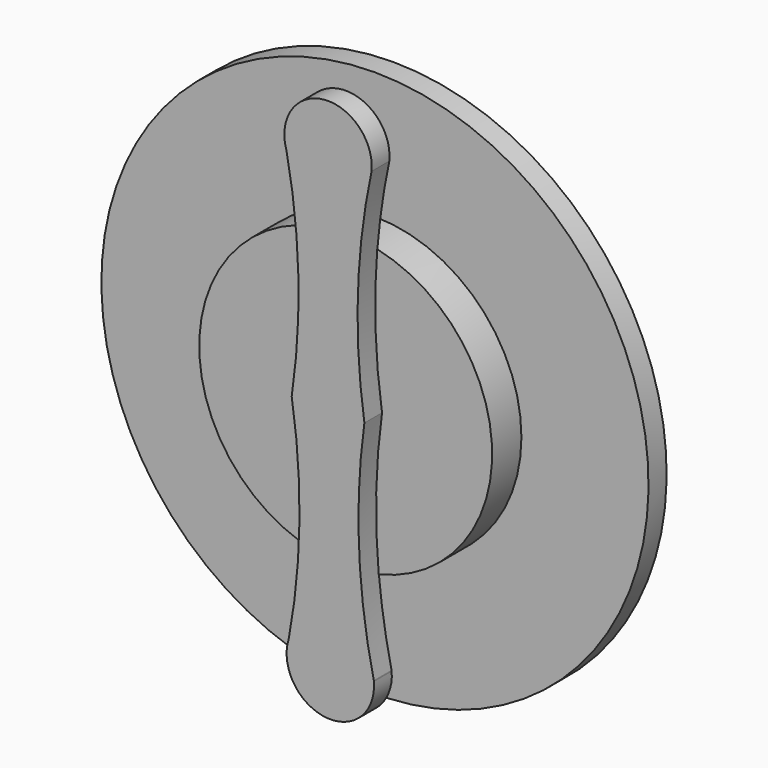
from build123d import *
from build123d import SkipClean  # not in build123d's __all__

# Parameters (mm, degrees)
F3_DEPTH = 25
F4_DEPTH = 9.7316764295
F5_R     = 2.7549652458
F6_DEPTH = 8.4777977318


with BuildPart() as f1:
    # F0 (on Right) → F1 (revolve)
    with BuildSketch(Plane.YZ):
        Polygon((0, 6.1400169507), (0, 8.2560488954), (0, 19.687499851), (-8.4777977318, 19.687499851), (-8.4777977318, 14.3298944458), (-25.8282721043, 14.3298944458), (-25.8282721043, 100.0597700477), (-35.5599485338, 100.0597700477), (-35.5599485338, 6.1400169507), align=None)
    revolve(axis=Axis((0, -24.406015873, 0), (0, -1, 0)))

    # F2 (on face) → F3 (cut)
    with BuildSketch(Plane.XZ.offset(35.5599485338)):
        with BuildLine():
            ThreePointArc((100.0597700477, 0), (77.1925232945, 63.6653118222), (19.0427553675, 98.2310085971))
            ThreePointArc((19.0427553675, 98.2310085971), (13.0501122552, 49.3824410014), (15.9002061052, 0.2502591582))
            ThreePointArc((15.9002061052, 0.2502591582), (13.5409533991, -48.9079370484), (20.0211640805, -97.6942178777))
            ThreePointArc((20.0211640805, -97.6942178777), (20.0382067589, -97.8618404932), (20.0537724887, -98.0296067062))
            ThreePointArc((20.0537724887, -98.0296067062), (77.5194602851, -63.2668227359), (100.0597700477, 0))
        make_face()
        with BuildLine():
            ThreePointArc((-18.1994950958, 94.1649181676), (-18.6134156028, 96.1995622705), (-19.0427553675, 98.2310085971))
            ThreePointArc((-19.0427553675, 98.2310085971), (-18.7317798871, 96.1750148827), (-18.1994950958, 94.1649181676))
        make_face()
        with BuildLine():
            ThreePointArc((-18.1994950958, 94.1649181676), (-18.7317798871, 96.1750148827), (-19.0427553675, 98.2310085971))
            ThreePointArc((-19.0427553675, 98.2310085971), (-100.058591646, -0.4856128205), (-18.0883946868, -98.4112166353))
            ThreePointArc((-18.0883946868, -98.4112166353), (-18.0761635611, -98.2428461722), (-18.0624471565, -98.0745901959))
            ThreePointArc((-18.0624471565, -98.0745901959), (-17.7720210603, -96.0155932105), (-17.2598383027, -94.0002806477))
            ThreePointArc((-17.2598383027, -94.0002806477), (-12.518858774, -47.0123005144), (-15.9239394561, 0.0913361759))
            ThreePointArc((-15.9239394561, 0.0913361759), (-12.9894678609, 47.2266312356), (-18.1994950958, 94.1649181676))
        make_face()
    extrude(amount=-F3_DEPTH, mode=Mode.SUBTRACT)

    # F2 (on face) → F4 (join, through all)
    with BuildSketch(Plane.XZ.offset(35.5599485338)):
        with BuildLine():
            ThreePointArc((15.9002061052, 0.2502591582), (13.0501122552, 49.3824410014), (19.0427553675, 98.2310085971))
            ThreePointArc((19.0427553675, 98.2310085971), (0, 119.1901359728), (-19.0427553675, 98.2310085971))
            ThreePointArc((-19.0427553675, 98.2310085971), (-18.6134156028, 96.1995622705), (-18.1994950958, 94.1649181676))
            ThreePointArc((-18.1994950958, 94.1649181676), (-12.9894678609, 47.2266312356), (-15.9239394561, 0.0913361759))
            ThreePointArc((-15.9239394561, 0.0913361759), (-12.518858774, -47.0123005144), (-17.2598383027, -94.0002806477))
            ThreePointArc((-17.2598383027, -94.0002806477), (-17.6534175167, -96.0389572316), (-18.0624471565, -98.0745901959))
            ThreePointArc((-18.0624471565, -98.0745901959), (1.1886840484, -118.8424860853), (20.0211640805, -97.6942178777))
            ThreePointArc((20.0211640805, -97.6942178777), (13.5409533991, -48.9079370484), (15.9002061052, 0.2502591582))
        make_face()
        with BuildLine():
            ThreePointArc((-18.1994950958, 94.1649181676), (-18.6134156028, 96.1995622705), (-19.0427553675, 98.2310085971))
            ThreePointArc((-19.0427553675, 98.2310085971), (-18.7317798871, 96.1750148827), (-18.1994950958, 94.1649181676))
        make_face()
        with BuildLine():
            ThreePointArc((-17.2598383027, -94.0002806477), (-17.7720210603, -96.0155932105), (-18.0624471565, -98.0745901959))
            ThreePointArc((-18.0624471565, -98.0745901959), (-17.6534175167, -96.0389572316), (-17.2598383027, -94.0002806477))
        make_face()
    with SkipClean():  # cleaning this boolean's faces spoils the solid; the shape is the same uncleaned
        extrude(amount=-F4_DEPTH)

    # F5 (on face) → F6 (join, through all)
    with BuildSketch(Plane(origin=(0, 0, 0), x_dir=(-1, 0, 0), z_dir=(0, 1, 0))):
        with BuildLine():
            ThreePointArc((5.24e-08, 19.687499851), (9.5966715729, 23.662571381), (13.5717430658, 33.2592429167))
            ThreePointArc((13.5717430658, 33.2592429167), (-9.5966715729, 42.8559144525), (5.24e-08, 19.687499851))
        make_face()
        with Locations((0, 33.2592429167)):
            Circle(F5_R, mode=Mode.SUBTRACT)
        with BuildLine():
            ThreePointArc((-15.2316062108, -16.6296214584), (-15.6940521066, -13.1169960083), (-17.0498748728, -9.8437501596))
            ThreePointArc((-17.0498748728, -9.8437501596), (-41.9126464465, -20.1422469085), (-15.2316062108, -16.6296214584))
        make_face()
        with Locations((-28.8033492765, -16.6296214584)):
            Circle(F5_R, mode=Mode.SUBTRACT)
        with BuildLine():
            ThreePointArc((42.3750923423, -16.6296214584), (32.3159749035, -3.5203243358), (17.0498750559, -9.8437498425))
            ThreePointArc((17.0498750559, -9.8437498425), (25.2907236496, -29.7389185809), (42.3750923423, -16.6296214584))
        make_face()
        with Locations((28.8033492765, -16.6296214584)):
            Circle(F5_R, mode=Mode.SUBTRACT)
    extrude(amount=-F6_DEPTH)

    # F7 (on Right) → F8 (revolve)
    with BuildSketch(Plane.YZ):
        Polygon((0, 12.1502038091), (0, 6.1231274158), (9.4215124846, 6.1231274158), (9.4215124846, 46.8469522893), (3.5086337011, 46.8469522893), (3.5086337011, 12.1502038091), align=None)
        Polygon((-25.9181205183, 64.11806494), (-25.9181205183, 21.7532776296), (-25.9181205183, 14.5246991888), (-8.9246770367, 14.5246991888), (-8.9246770367, 18.3331295848), (-13.284237124, 18.3331295848), (-13.284237124, 57.3514103889), (0, 57.3514103889), (0, 119.7736561298), (-9.902862832, 119.7736561298), (-9.902862832, 64.11806494), align=None)
    revolve(axis=Axis((0, -24.5498530567, 0), (0, -1, 0)))


solid = f1.part
